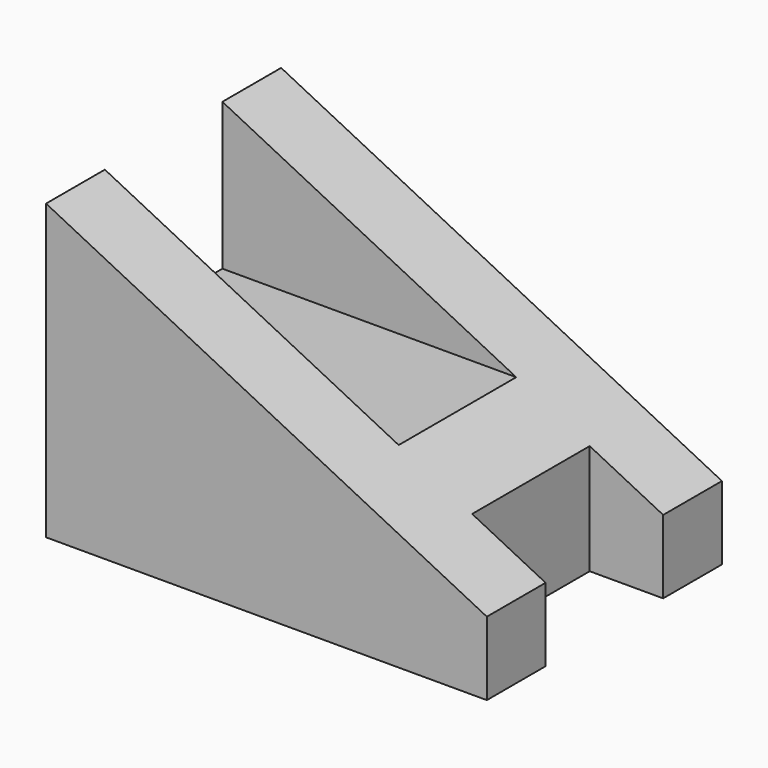
from build123d import *

# Parameters (mm, degrees)
F1_DEPTH = 10
F2_W     = 10
F2_H     = 20
F3_DEPTH = 56
F4_W     = 10
F4_H     = 10
F5_REACH = 34.1431356237


# Not quite as in the source:
# - an extrude ends at something that could not be found from the text; its depth is read off the source's solid


with BuildPart() as f1:
    # F0 (on Front) → F1 (new body, symmetric)
    with BuildSketch(Plane.XZ):
        Polygon((0, 20), (0, 0), (30, 0), (30, 5), align=None)
    extrude(amount=F1_DEPTH, both=True)

    # F2 (on face) → F3 (cut, through all)
    with BuildSketch(Plane(origin=(0, 0, 0), x_dir=(0, -1, 0), z_dir=(-1, 0, 0))):
        with Locations((0, 20)):
            Rectangle(F2_W, F2_H)
    extrude(amount=-F3_DEPTH, mode=Mode.SUBTRACT)

    f5_end = Plane(origin=(17.5, 0, 11.25), x_dir=(0.894427191, 0, -0.4472135955), z_dir=(0.4472135955, 0, 0.894427191))
    # F4 (on face) → F5 (cut, up to a plane its end follows)
    with BuildSketch(Plane(origin=(0, 0, 0), x_dir=(1, 0, 0), z_dir=(0, 0, -1))):
        with Locations((30, 0)):
            Rectangle(F4_W, F4_H)
    f5_long = extrude(amount=-F5_REACH, mode=Mode.PRIVATE)
    add(split(f5_long, bisect_by=f5_end, keep=Keep.BOTTOM, mode=Mode.PRIVATE), mode=Mode.SUBTRACT)


solid = f1.part
